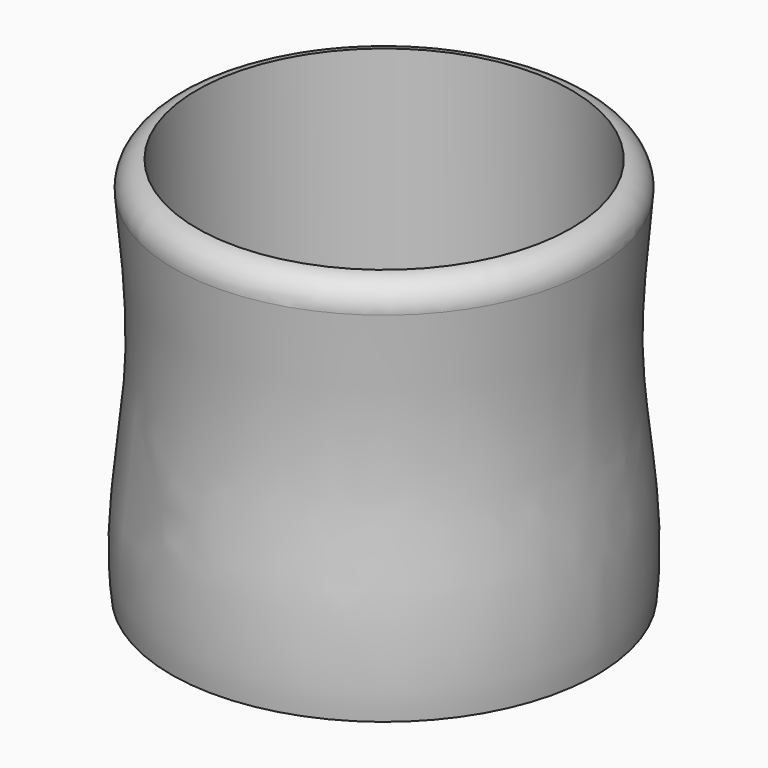
from build123d import *

# Parameters (mm, degrees)
F4_DEPTH = 1
F6_DEPTH = 75


# Not quite as in the source:
# - a fillet or chamfer that OpenCascade refuses, or shapes differently, is made with other operations: its cross-section is extruded or revolved along the edge and cut away or added


with BuildPart() as f1:
    # F0 (on Front) → F1 (revolve)
    with BuildSketch(Plane.XZ):
        with BuildLine():
            Line((36.5, 0), (36.5, -36))
            Line((36.5, -36), (0, -36))
            Line((0, -36), (0, -39))
            Line((0, -39), (36.5, -39))
            Line((36.5, -39), (41.5, -39))
            add(Edge.make_bspline(
                [(41.5, 36), (40.5130405729, 24.1204033311), (37.2400196897, -0.6601610616), (43.1067779162, -24.7504109869), (41.5, -39)],
                knots=[0, 0, 0, 0, 0.4900244398, 1, 1, 1, 1], degree=3))
            Line((41.5, 36), (36.5, 36))
            Line((36.5, 36), (36.5, 0))
        make_face()
    revolve(axis=Axis((0, 0, -37.5), (0, 0, -1)))

    # F2: fillet of radius 5 on 1 edges, made by hand

    # F2_s1 → F2_t2 (revolve, cut)
    with BuildSketch(Plane.XZ):
        with BuildLine():
            ThreePointArc((36.5, 36), (39.8850667362, 34.2149523953), (41.0164086347, 30.5591163393))
            Line((41.0164086347, 30.5591163393), (41.1159802932, 30.5498705395))
            ThreePointArc((41.1159802932, 30.5498705395), (41.3643970641, 33.2700710676), (41.5996566603, 35.9917205034))
            Line((41.5996566603, 35.9917205034), (41.5, 36.1))
            ThreePointArc((41.5, 36.1), (39, 36.1), (36.5092434859, 36.0995718734))
            Line((36.5092434859, 36.0995718734), (36.5, 36))
        make_face()
    revolve(axis=Axis((0, 0, 36), (0, 0, -1)), mode=Mode.SUBTRACT)

    # F3 (on face) → F4 (cut)
    with BuildSketch(Plane(origin=(0, 0, -39), x_dir=(1, 0, 0), z_dir=(0, 0, -1))):
        with BuildLine():
            ThreePointArc((41.5, 0), (41.4936223113, 0.7275352131), (41.4744912055, 1.4548468121))
            Line((41.4744912055, 1.4548468121), (39.5, 1.4548468121))
            Line((39.5, 1.4548468121), (39.5, -1.5451531879))
            Line((39.5, -1.5451531879), (41.4712249834, -1.5451531879))
            ThreePointArc((41.4712249834, -1.5451531879), (41.4928056223, -0.7727105499), (41.5, 0))
        make_face()
    extrude(amount=-F4_DEPTH, mode=Mode.SUBTRACT)

    # F5 (on face) → F6 (cut, symmetric)
    with BuildSketch(Plane.XY.offset(-36)):
        with BuildLine():
            ThreePointArc((-2.5, 25.4165305825), (-4.5062959033, 29.4212447772), (-8.9150943126, 30.2121022989))
            ThreePointArc((-8.9150943126, 30.2121022989), (-22.2738639656, 22.2738639656), (-30.2121022989, 8.9150943126))
            ThreePointArc((-30.2121022989, 8.9150943126), (-29.4212447772, 4.5062959033), (-25.4165305825, 2.5))
            Line((-25.4165305825, 2.5), (-7.5, 2.5))
            ThreePointArc((-7.5, 2.5), (-3.9644660941, 3.9644660941), (-2.5, 7.5))
            Line((-2.5, 7.5), (-2.5, 25.4165305825))
        make_face()
        with BuildLine():
            ThreePointArc((-8.9150943126, -30.2121022989), (-4.5062959033, -29.4212447772), (-2.5, -25.4165305825))
            Line((-2.5, -25.4165305825), (-2.5, -7.5))
            ThreePointArc((-2.5, -7.5), (-3.9644660941, -3.9644660941), (-7.5, -2.5))
            Line((-7.5, -2.5), (-25.4165305825, -2.5))
            ThreePointArc((-25.4165305825, -2.5), (-29.4212447772, -4.5062959033), (-30.2121022989, -8.9150943126))
            ThreePointArc((-30.2121022989, -8.9150943126), (-22.2738639656, -22.2738639656), (-8.9150943126, -30.2121022989))
        make_face()
        with BuildLine():
            ThreePointArc((30.2121022989, -8.9150943126), (29.4212447772, -4.5062959033), (25.4165305825, -2.5))
            Line((25.4165305825, -2.5), (7.5, -2.5))
            ThreePointArc((7.5, -2.5), (3.9644660941, -3.9644660941), (2.5, -7.5))
            Line((2.5, -7.5), (2.5, -25.4165305825))
            ThreePointArc((2.5, -25.4165305825), (4.5062959033, -29.4212447772), (8.9150943126, -30.2121022989))
            ThreePointArc((8.9150943126, -30.2121022989), (22.2738639656, -22.2738639656), (30.2121022989, -8.9150943126))
        make_face()
        with BuildLine():
            ThreePointArc((8.9150943126, 30.2121022989), (4.5062959033, 29.4212447772), (2.5, 25.4165305825))
            Line((2.5, 25.4165305825), (2.5, 7.5))
            ThreePointArc((2.5, 7.5), (3.9644660941, 3.9644660941), (7.5, 2.5))
            Line((7.5, 2.5), (25.4165305825, 2.5))
            ThreePointArc((25.4165305825, 2.5), (29.4212447772, 4.5062959033), (30.2121022989, 8.9150943126))
            ThreePointArc((30.2121022989, 8.9150943126), (22.2738639656, 22.2738639656), (8.9150943126, 30.2121022989))
        make_face()
    extrude(amount=F6_DEPTH, both=True, mode=Mode.SUBTRACT)


solid = f1.part
